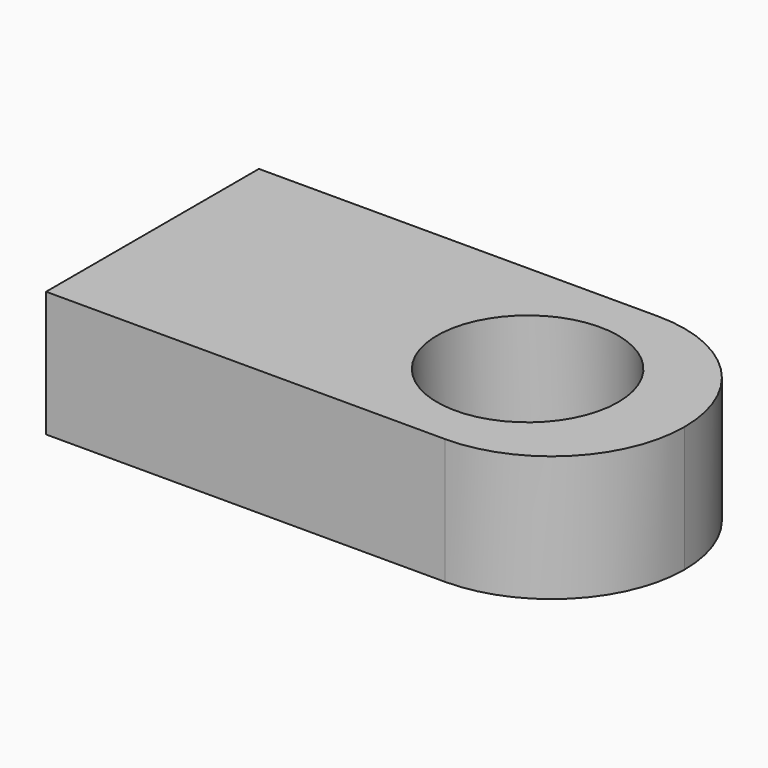
from build123d import *

# Parameters (mm, degrees)
F0_W     = 12.7
F0_H     = 6.35
F1_DEPTH = 3
F3_R     = 3.17499
F2_R     = 2.159
F4_DEPTH = 25.4


# Not quite as in the source:
# - a fillet or chamfer is up to 0.001 mm smaller than in the source, because OpenCascade refuses the exact size


with BuildPart() as f1:
    # F0 (on Top) → F1 (new body)
    with BuildSketch(Plane.XY):
        with Locations((6.35, 3.175)):
            Rectangle(F0_W, F0_H)
    extrude(amount=F1_DEPTH)

    # F3 (radius 3.175 in the source; OpenCascade refuses exactly that, so slightly less here)
    f3_edges = [f1.edges().sort_by_distance(p)[0] for p in [
        (12.7, 6.35, 1.5),
        (12.7, 0, 1.5),
    ]]
    fillet(f3_edges, radius=F3_R)

    # F2 (on face) → F4 (cut)
    with BuildSketch(Plane.XY.offset(3)):
        with Locations((8.9535, 3.175)):
            Circle(F2_R)
    extrude(amount=-F4_DEPTH, mode=Mode.SUBTRACT)


solid = f1.part
